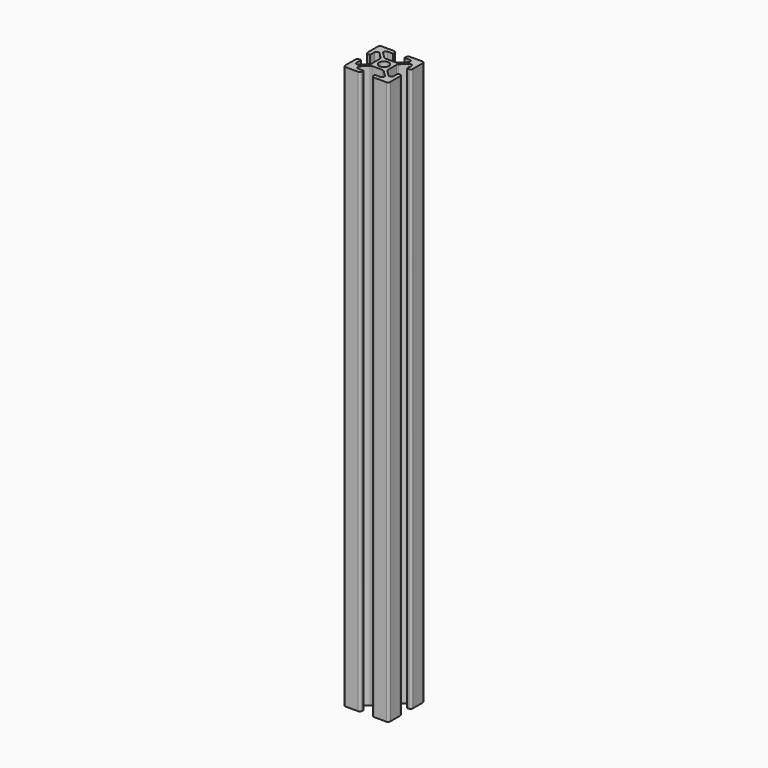
from build123d import *

# Parameters (mm, degrees)
F0_R     = 2.15
F1_DEPTH = 250


# Not quite as in the source:
# - ends of sketch curves that miss each other by under 0.0002 mm in the source are joined


with BuildPart() as f1:
    # F0 (on Top) → F1 (new body)
    with BuildSketch(Plane.XY):
        with BuildLine():
            Line((10, 3.5), (10, 9))
            ThreePointArc((10, 9), (9.7071067812, 9.7071067812), (9, 10))
            Line((9, 10), (3.5, 10))
            ThreePointArc((3.5, 10), (2.7928932188, 9.7071067812), (2.5, 9))
            Line((2.5, 9), (2.5, 8.2))
            Line((2.5, 8.2), (4.9, 8.2))
            ThreePointArc((4.9, 8.2), (5.8238795325, 7.5826834324), (5.6071067812, 6.4928932188))
            Line((5.6071067812, 6.4928932188), (3.057107, 3.942893))
            ThreePointArc((3.057107, 3.942893), (2.7326834324, 3.7261204675), (2.35, 3.65))
            Line((2.35, 3.65), (-2.35, 3.65))
            ThreePointArc((-2.35, 3.65), (-2.7326834324, 3.7261204675), (-3.0571067812, 3.9428932188))
            Line((-3.0571067812, 3.9428932188), (-5.607107, 6.492893))
            ThreePointArc((-5.607107, 6.492893), (-5.8238795325, 7.5826834324), (-4.9, 8.2))
            Line((-4.9, 8.2), (-2.5, 8.2))
            Line((-2.5, 8.2), (-2.5, 9))
            ThreePointArc((-2.5, 9), (-2.7928932188, 9.7071067812), (-3.5, 10))
            Line((-3.5, 10), (-9, 10))
            ThreePointArc((-9, 10), (-9.7071067812, 9.7071067812), (-10, 9))
            Line((-10, 9), (-10, 3.5))
            ThreePointArc((-10, 3.5), (-9.7071067812, 2.7928932188), (-9, 2.5))
            Line((-9, 2.5), (-8.2, 2.5))
            Line((-8.2, 2.5), (-8.2, 4.9))
            ThreePointArc((-8.2, 4.9), (-7.5826834324, 5.8238795325), (-6.4928932188, 5.6071067812))
            Line((-6.4928932188, 5.6071067812), (-3.942893, 3.057107))
            ThreePointArc((-3.942893, 3.057107), (-3.7261204675, 2.7326834324), (-3.65, 2.35))
            Line((-3.65, 2.35), (-3.65, -2.35))
            ThreePointArc((-3.65, -2.35), (-3.7261204675, -2.7326834324), (-3.9428932188, -3.0571067812))
            Line((-3.9428932188, -3.0571067812), (-6.492893, -5.607107))
            ThreePointArc((-6.492893, -5.607107), (-7.5826834324, -5.8238795325), (-8.2, -4.9))
            Line((-8.2, -4.9), (-8.2, -2.5))
            Line((-8.2, -2.5), (-9, -2.5))
            ThreePointArc((-9, -2.5), (-9.7071067812, -2.7928932188), (-10, -3.5))
            Line((-10, -3.5), (-10, -9))
            ThreePointArc((-10, -9), (-9.7071067812, -9.7071067812), (-9, -10))
            Line((-9, -10), (-3.5, -10))
            ThreePointArc((-3.5, -10), (-2.7928932188, -9.7071067812), (-2.5, -9))
            Line((-2.5, -9), (-2.5, -8.2))
            Line((-2.5, -8.2), (-4.9, -8.2))
            ThreePointArc((-4.9, -8.2), (-5.8238795325, -7.5826834324), (-5.6071067812, -6.4928932188))
            Line((-5.6071067812, -6.4928932188), (-3.057107, -3.942893))
            ThreePointArc((-3.057107, -3.942893), (-2.7326834324, -3.7261204675), (-2.35, -3.65))
            Line((-2.35, -3.65), (2.35, -3.65))
            ThreePointArc((2.35, -3.65), (2.7326834324, -3.7261204675), (3.0571067812, -3.9428932188))
            Line((3.0571067812, -3.9428932188), (5.607107, -6.492893))
            ThreePointArc((5.607107, -6.492893), (5.8238795325, -7.5826834324), (4.9, -8.2))
            Line((4.9, -8.2), (2.5, -8.2))
            Line((2.5, -8.2), (2.5, -9))
            ThreePointArc((2.5, -9), (2.7928932188, -9.7071067812), (3.5, -10))
            Line((3.5, -10), (9, -10))
            ThreePointArc((9, -10), (9.7071067812, -9.7071067812), (10, -9))
            Line((10, -9), (10, -3.5))
            ThreePointArc((10, -3.5), (9.7071067812, -2.7928932188), (9, -2.5))
            Line((9, -2.5), (8.2, -2.5))
            Line((8.2, -2.5), (8.2, -4.9))
            ThreePointArc((8.2, -4.9), (7.5826834324, -5.8238795325), (6.4928932188, -5.6071067812))
            Line((6.4928932188, -5.6071067812), (3.942893, -3.057107))
            ThreePointArc((3.942893, -3.057107), (3.7261204675, -2.7326834324), (3.65, -2.35))
            Line((3.65, -2.35), (3.65, 2.35))
            ThreePointArc((3.65, 2.35), (3.7261204675, 2.7326834324), (3.9428932188, 3.0571067812))
            Line((3.9428932188, 3.0571067812), (6.492893, 5.607107))
            ThreePointArc((6.492893, 5.607107), (7.5826834324, 5.8238795325), (8.2, 4.9))
            Line((8.2, 4.9), (8.2, 2.5))
            Line((8.2, 2.5), (9, 2.5))
            ThreePointArc((9, 2.5), (9.7071067812, 2.7928932188), (10, 3.5))
        make_face()
        Circle(F0_R, mode=Mode.SUBTRACT)
    extrude(amount=F1_DEPTH)


solid = f1.part
